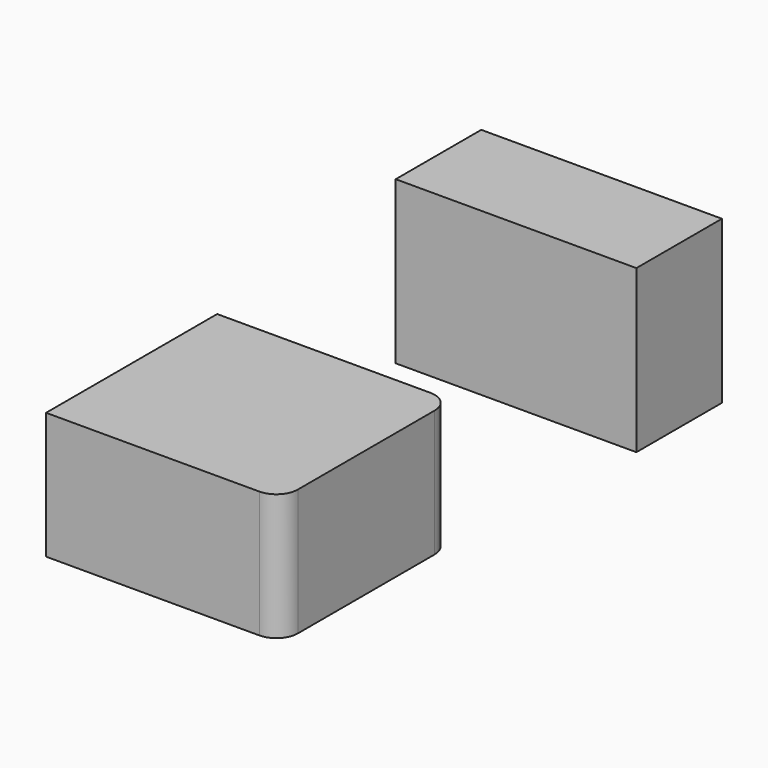
from build123d import *

# Parameters (mm, degrees)
F0_W     = 55.7312387973
F0_H     = 30.0914160907
F1_DEPTH = 25.4
F2_DEPTH = 25.4
F3_R     = 5.08


with BuildPart() as f1:
    # F0 (on Front) → F1 (new body)
    with BuildSketch(Plane.XZ):
        with Locations((18.7620026991, 4.2443163693)):
            Rectangle(F0_W, F0_H)
    extrude(amount=F1_DEPTH)

    # F2 (add): a face of the model
    f2_faces = [f1.faces().sort_by_distance(p)[0] for p in [
        (18.7620026991, -25.4, 4.2443163693),
    ]]
    extrude(f2_faces, amount=F2_DEPTH)

    # F3
    f3_edges = [f1.edges().sort_by_distance(p)[0] for p in [
        (46.627622, -50.8, 4.244316),
        (46.627622, 0, 4.244316),
    ]]
    fillet(f3_edges, radius=F3_R)


with BuildPart() as f1b:
    # F0 (on Front) → F1, piece 2 (new body)
    with BuildSketch(Plane.XZ):
        Polygon((53.6285489798, 78.2144851983), (53.6285489798, 54.7660994999), (53.6285489798, 39.709392935), (110.8027845621, 39.709392935), (110.8027845621, 78.2144851983), align=None)
    extrude(amount=F1_DEPTH)


solid = Compound([f1.part, f1b.part])
